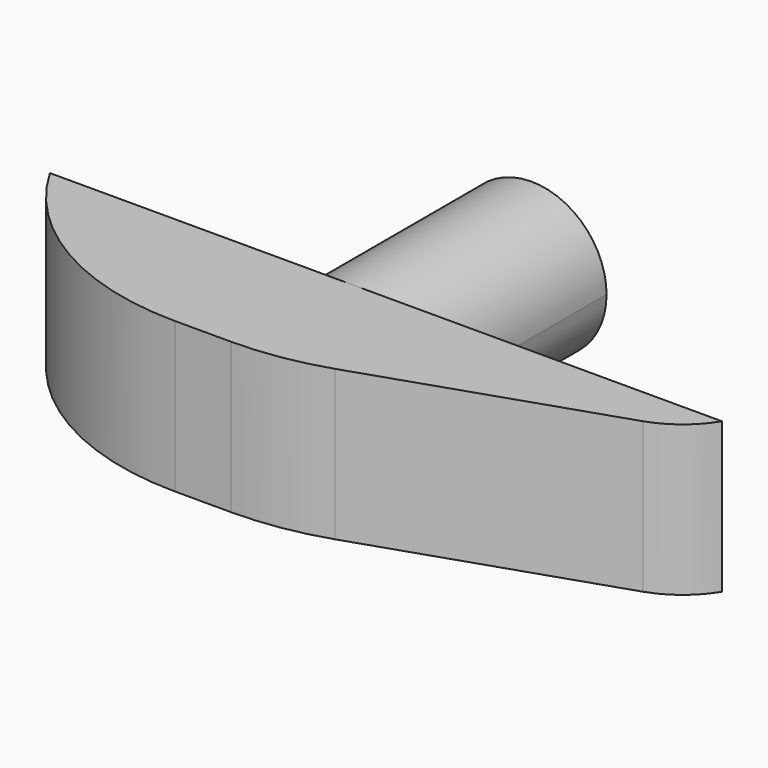
from build123d import *

# Parameters (mm, degrees)
F1_DEPTH    = 10
F2_DEPTH    = 6
F3_SIZE2    = 15
F3_SIZE     = 5
F4_T1_DEPTH = 58.6615242271
F5_R        = 13
F6_T1_DEPTH = 18.0508625467


# Not quite as in the source:
# - a fillet or chamfer that OpenCascade refuses, or shapes differently, is made with other operations: its cross-section is extruded or revolved along the edge and cut away or added


with BuildPart() as f1:
    # F0 (on Front) → F1 (new body)
    with BuildSketch(Plane.XZ):
        with BuildLine():
            ThreePointArc((2.15, -0.0081778196), (-3.4744734584, 2.4513486566), (-1.4615047685, -3.3479555451))
            Line((-1.4615047685, -3.3479555451), (-0.9384952315, -3.3479555451))
            ThreePointArc((-0.9384952315, -3.3479555451), (1.2595264762, -2.2826512779), (2.15, -0.0081778196))
        make_face()
    extrude(amount=-F1_DEPTH)

    # F0 (on Front) → F2 (join)
    with BuildSketch(Plane.XZ):
        with BuildLine():
            Line((15.3, 3.3520444549), (-14.7, 3.3520444549))
            Line((-14.7, 3.3520444549), (-14.7, -3.3479555451))
            Line((-14.7, -3.3479555451), (-1.4615047685, -3.3479555451))
            ThreePointArc((-1.4615047685, -3.3479555451), (-3.4744734584, 2.4513486566), (2.15, -0.0081778196))
            ThreePointArc((2.15, -0.0081778196), (1.2595264762, -2.2826512779), (-0.9384952315, -3.3479555451))
            Line((-0.9384952315, -3.3479555451), (15.3, -3.3479555451))
            Line((15.3, -3.3479555451), (15.3, 3.3520444549))
        make_face()
        with BuildLine():
            ThreePointArc((2.15, -0.0081778196), (-3.4744734584, 2.4513486566), (-1.4615047685, -3.3479555451))
            Line((-1.4615047685, -3.3479555451), (-0.9384952315, -3.3479555451))
            ThreePointArc((-0.9384952315, -3.3479555451), (1.2595264762, -2.2826512779), (2.15, -0.0081778196))
        make_face()
    extrude(amount=F2_DEPTH)

    # F3
    f3_edges = [f1.edges().sort_by_distance(p)[0] for p in [
        (15.3, -6, 0.002044),
    ]]
    f3_side = f1.faces().sort_by_distance((15.3, -3, 0.002044))[0]
    chamfer(f3_edges, length=F3_SIZE, length2=F3_SIZE2, reference=f3_side)

    # F4: fillet of radius 12 on 1 edges, made by hand

    # F4_s2 → F4_t1 (cut)
    with BuildSketch(Plane.XY.offset(-29.3287176586)):
        with BuildLine():
            ThreePointArc((-4.3076951546, -6), (-10.3076951546, -4.3923048454), (-14.7, 0))
            Line((-14.7, 0), (-14.7, -6))
            Line((-14.7, -6), (-4.3076951546, -6))
        make_face()
    extrude(amount=F4_T1_DEPTH, mode=Mode.SUBTRACT)

    # F5
    f5_edges = [f1.edges().sort_by_distance(p)[0] for p in [
        (0.3, -6, 0.002044),
    ]]
    fillet(f5_edges, radius=F5_R)

    # F6: fillet of radius 4 on 1 edges, made by hand

    # F6_s2 → F6_t1 (cut)
    with BuildSketch(Plane.XY.offset(-9.0233868185)):
        with BuildLine():
            ThreePointArc((13.1463252567, -1.7178915811), (14.3757224349, -1.0502059409), (15.3, 0))
            Line((15.3, 0), (15.3, -1))
            Line((15.3, -1), (13.1463252567, -1.7178915811))
        make_face()
    extrude(amount=F6_T1_DEPTH, mode=Mode.SUBTRACT)


solid = f1.part
